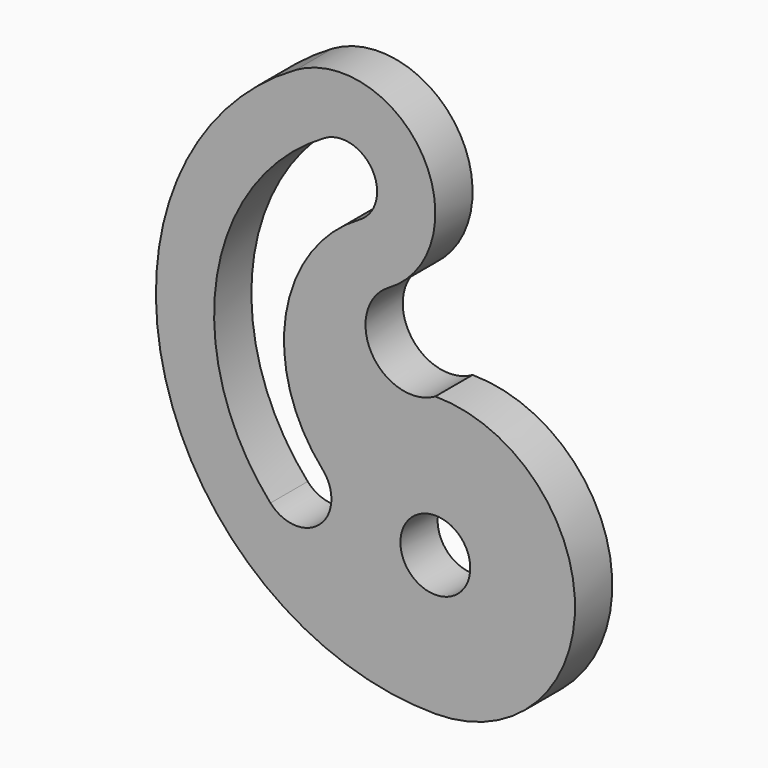
from build123d import *

# Parameters (mm, degrees)
F0_R     = 190.5
F1_DEPTH = 254


# Not quite as in the source:
# - ends of sketch curves that miss each other by under 0.0002 mm in the source are joined


with BuildPart() as f1:
    # F0 (on Front) → F1 (new body)
    with BuildSketch(Plane.XZ):
        with BuildLine():
            ThreePointArc((-253.9996830053, 1201.9410881396), (-68.0591863861, 1895.8819687424), (-762, 2081.8227153675))
            ThreePointArc((-762, 2081.8227153675), (-1472.0709592645, 367.5597752638), (0, -762))
            ThreePointArc((0, -762), (761.9891288024, -7.75e-08), (0, 761.9999998449))
            ThreePointArc((0, 761.9999998449), (-346.9703855723, 854.9707025672), (-253.9996830053, 1201.9410881396))
        make_face()
        Circle(F0_R, mode=Mode.SUBTRACT)
        with BuildLine():
            ThreePointArc((-603.25, 1806.8596496659), (-343.0221605791, 1737.131810245), (-412.75, 1476.9039708241))
            ThreePointArc((-412.75, 1476.9039708241), (-815.1218466146, 892.4861122222), (-615.2913719088, 211.666666422))
            ThreePointArc((-615.2913719088, 211.666666422), (-630.28168848, -57.3236501492), (-899.2720050513, -42.333333578))
            ThreePointArc((-899.2720050513, -42.333333578), (-1191.3319294955, 952.7104717353), (-603.25, 1806.8596496659))
        make_face(mode=Mode.SUBTRACT)
    extrude(amount=F1_DEPTH)


solid = f1.part
